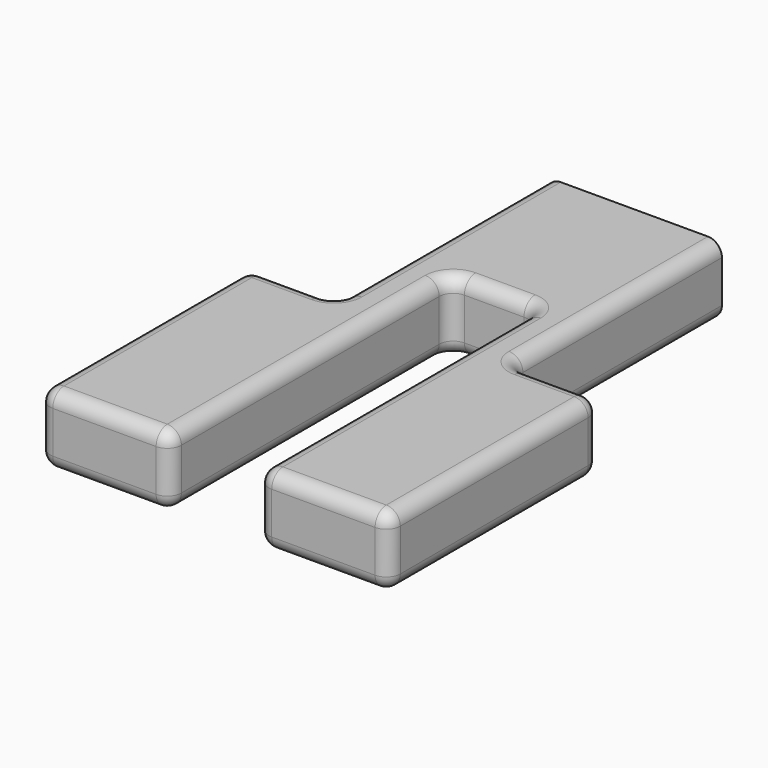
from build123d import *

# Parameters (mm, degrees)
F1_DEPTH = 25.4
F2_R     = 5.08


with BuildPart() as f1:
    # F0 (on Top) → F1 (new body)
    with BuildSketch(Plane.XY):
        Polygon((14.8781485382, 63.5), (-48.6218514618, 63.5), (-48.6218514618, -31.75), (-80.3718514618, -31.75), (-80.3718514618, -127), (-32.7468514618, -127), (-32.7468514618, 0), (-0.9968514618, 0), (-0.9968514618, -127), (46.6281485382, -127), (46.6281485382, -31.75), (14.8781485382, -31.75), align=None)
    extrude(amount=F1_DEPTH)

    # F2
    f2_edges = [f1.edges().sort_by_distance(p)[0] for p in [
        (14.878149, 15.875, 25.4),
        (-48.621851, 15.875, 25.4),
        (-48.621851, 15.875, 0),
        (14.878149, 15.875, 0),
        (14.878149, -31.75, 12.7),
        (-48.621851, -31.75, 12.7),
        (-80.371851, -31.75, 12.7),
        (-80.371851, -79.375, 25.4),
        (-80.371851, -79.375, 0),
        (-56.559351, -127, 25.4),
        (-80.371851, -127, 12.7),
        (22.815649, -127, 25.4),
        (46.628149, -79.375, 25.4),
        (-0.996851, -127, 12.7),
        (46.628149, -127, 12.7),
        (22.815649, -127, 0),
        (-32.746851, -127, 12.7),
        (-16.871851, 0, 25.4),
        (-32.746851, -63.5, 25.4),
        (-0.996851, -63.5, 25.4),
        (46.628149, -31.75, 12.7),
        (-0.996851, -63.5, 0),
        (-16.871851, 0, 0),
        (46.628149, -79.375, 0),
        (-32.746851, -63.5, 0),
        (-0.996851, 0, 12.7),
        (-32.746851, 0, 12.7),
        (-56.559351, -127, 0),
        (-64.496851, -31.75, 0),
        (-64.496851, -31.75, 25.4),
        (30.753149, -31.75, 0),
        (30.753149, -31.75, 25.4),
    ]]
    fillet(f2_edges, radius=F2_R)


solid = f1.part
